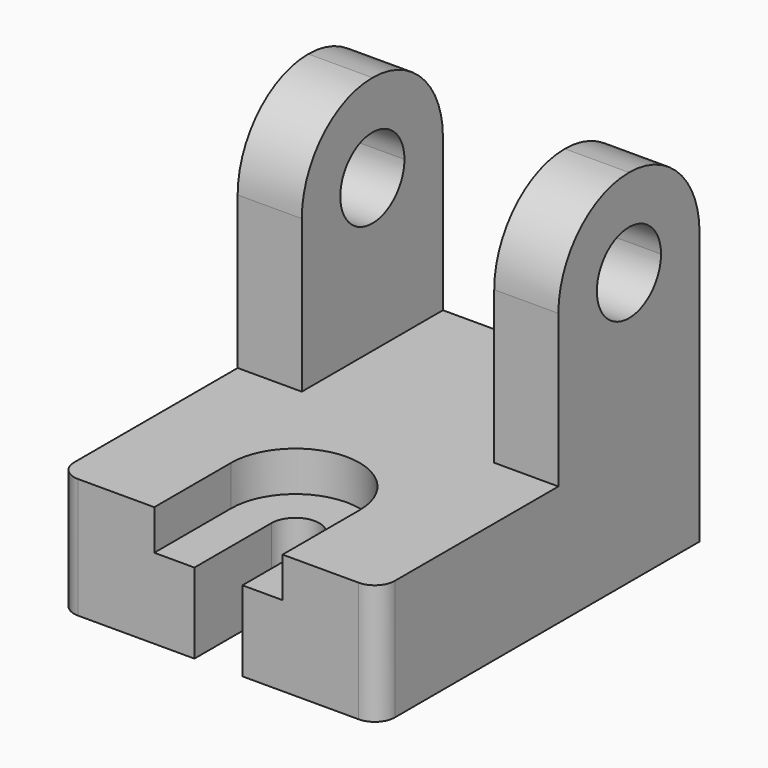
from build123d import *

# Parameters (mm, degrees)
F1_DEPTH = 100
F0_W     = 16
F0_H     = 60
F2_DEPTH = 44
F3_R     = 5
F4_R     = 21.99999
F6_DEPTH = 80
F8_DEPTH = 30
F9_DEPTH = 10


# Not quite as in the source:
# - a fillet or chamfer is up to 0.001 mm smaller than in the source, because OpenCascade refuses the exact size


with BuildPart() as f1:
    # F0 (on Front) → F1 (new body)
    with BuildSketch(Plane.XZ):
        Polygon((0, 30), (0, 0), (80, 0), (80, 30), (64, 30), (16, 30), align=None)
    extrude(amount=F1_DEPTH)

    # F0 (on Front) → F2 (join)
    with BuildSketch(Plane.XZ):
        with Locations((8, 60)):
            Rectangle(F0_W, F0_H)
        with Locations((72, 60)):
            Rectangle(F0_W, F0_H)
    extrude(amount=F2_DEPTH)

    # F3
    f3_edges = [f1.edges().sort_by_distance(p)[0] for p in [
        (80, -100, 15),
        (0, -100, 15),
    ]]
    fillet(f3_edges, radius=F3_R)

    # F4 (radius 22 in the source; OpenCascade refuses exactly that, so slightly less here)
    f4_edges = [f1.edges().sort_by_distance(p)[0] for p in [
        (72, -44, 90),
        (72, 0, 90),
        (8, 0, 90),
        (8, -44, 90),
    ]]
    fillet(f4_edges, radius=F4_R)

    # F5 (on face) → F6 (cut)
    with BuildSketch(Plane.YZ.offset(80)):
        with BuildLine():
            Line((-32, 68), (-22, 68))
            Line((-22, 68), (-22, 78))
            ThreePointArc((-22, 78), (-29.0710678119, 75.0710678119), (-32, 68))
        make_face()
        with BuildLine():
            Line((-22, 78), (-22, 68))
            Line((-22, 68), (-12, 68))
            ThreePointArc((-12, 68), (-14.9289321881, 75.0710678119), (-22, 78))
        make_face()
        with BuildLine():
            Line((-12, 68), (-22, 68))
            Line((-22, 68), (-32, 68))
            ThreePointArc((-32, 68), (-22, 58), (-12, 68))
        make_face()
    extrude(amount=-F6_DEPTH, mode=Mode.SUBTRACT)

    # F7 (on face) → F8 (cut)
    with BuildSketch(Plane.XY.offset(30)):
        with BuildLine():
            Line((40, -92), (40, -100))
            Line((40, -100), (45.9878519068, -100))
            Line((45.9878519068, -100), (45.9878519068, -90.8373053329))
            ThreePointArc((45.9878519068, -90.8373053329), (43.0498454611, -91.7066368986), (40, -92))
        make_face()
        with BuildLine():
            Line((34.0121480932, -100), (40, -100))
            Line((40, -100), (40, -92))
            ThreePointArc((40, -92), (36.9501545389, -91.7066368986), (34.0121480932, -90.8373053329))
            Line((34.0121480932, -90.8373053329), (34.0121480932, -100))
        make_face()
        with BuildLine():
            Line((40, -81.9878519068), (40, -92))
            ThreePointArc((40, -92), (43.0498454611, -91.7066368986), (45.9878519068, -90.8373053329))
            Line((45.9878519068, -90.8373053329), (45.9878519068, -76))
            ThreePointArc((45.9878519068, -76), (44.234050688, -80.234050688), (40, -81.9878519068))
        make_face()
        with BuildLine():
            ThreePointArc((34.0121480932, -90.8373053329), (36.9501545389, -91.7066368986), (40, -92))
            Line((40, -92), (40, -81.9878519068))
            ThreePointArc((40, -81.9878519068), (35.765949312, -80.234050688), (34.0121480932, -76))
            Line((34.0121480932, -76), (34.0121480932, -90.8373053329))
        make_face()
        with BuildLine():
            ThreePointArc((34.0121480932, -76), (35.765949312, -80.234050688), (40, -81.9878519068))
            ThreePointArc((40, -81.9878519068), (44.234050688, -80.234050688), (45.9878519068, -76))
            ThreePointArc((45.9878519068, -76), (40, -70.0121480932), (34.0121480932, -76))
        make_face()
    extrude(amount=-F8_DEPTH, mode=Mode.SUBTRACT)

    # F7 (on face) → F9 (cut)
    with BuildSketch(Plane.XY.offset(30)):
        with BuildLine():
            ThreePointArc((24, -76), (26.7371641323, -84.9497030535), (34.0121480932, -90.8373053329))
            Line((34.0121480932, -90.8373053329), (34.0121480932, -76))
            ThreePointArc((34.0121480932, -76), (40, -70.0121480932), (45.9878519068, -76))
            Line((45.9878519068, -76), (45.9878519068, -90.8373053329))
            ThreePointArc((45.9878519068, -90.8373053329), (53.2628358677, -84.9497030535), (56, -76))
            ThreePointArc((56, -76), (40, -60), (24, -76))
        make_face()
        with BuildLine():
            Line((24, -100), (34.0121480932, -100))
            Line((34.0121480932, -100), (34.0121480932, -90.8373053329))
            ThreePointArc((34.0121480932, -90.8373053329), (26.7371641323, -84.9497030535), (24, -76))
            Line((24, -76), (24, -100))
        make_face()
        with BuildLine():
            Line((45.9878519068, -90.8373053329), (45.9878519068, -100))
            Line((45.9878519068, -100), (56, -100))
            Line((56, -100), (56, -76))
            ThreePointArc((56, -76), (53.2628358677, -84.9497030535), (45.9878519068, -90.8373053329))
        make_face()
    extrude(amount=-F9_DEPTH, mode=Mode.SUBTRACT)


solid = f1.part
